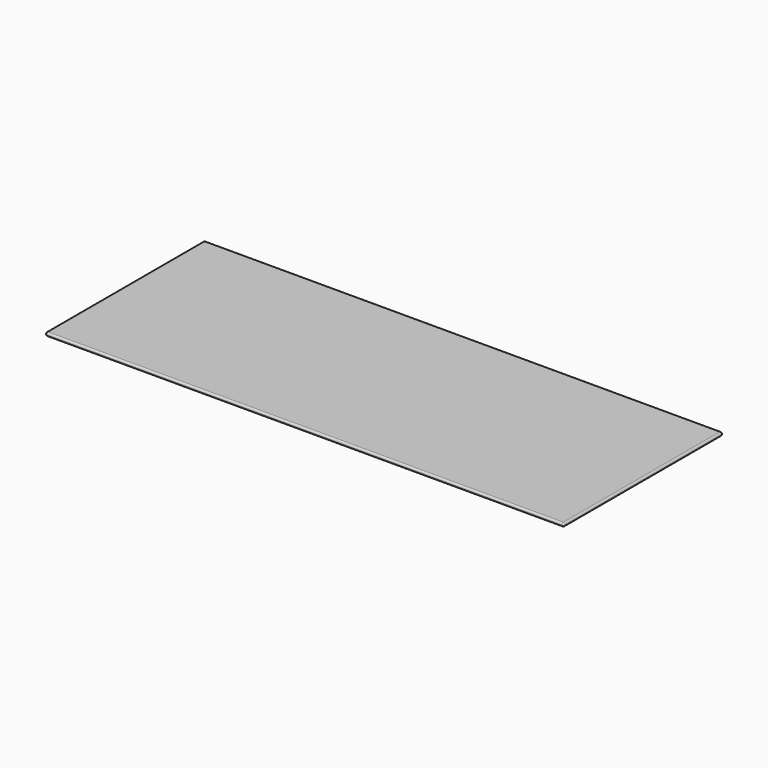
from build123d import *

# Parameters (mm, degrees)
F0_W     = 148.2852
F0_H     = 56.896
F1_DEPTH = 1.016
F2_R     = 0.50799


# Not quite as in the source:
# - a fillet or chamfer is up to 0.001 mm smaller than in the source, because OpenCascade refuses the exact size


with BuildPart() as f1:
    # F0 (on Top) → F1 (new body)
    with BuildSketch(Plane.XY):
        Rectangle(F0_W, F0_H)
    extrude(amount=F1_DEPTH)

    # F2 (radius 0.508 in the source; OpenCascade refuses exactly that, so slightly less here)
    f2_edges = [f1.edges().sort_by_distance(p)[0] for p in [
        (-74.1426, -28.448, 0.508),
        (74.1426, -28.448, 0.508),
        (0, -28.448, 0),
        (0, -28.448, 1.016),
        (-74.1426, 28.448, 0.508),
        (-74.1426, 0, 0),
        (-74.1426, 0, 1.016),
        (74.1426, 28.448, 0.508),
        (0, 28.448, 0),
        (0, 28.448, 1.016),
        (74.1426, 0, 0),
        (74.1426, 0, 1.016),
    ]]
    fillet(f2_edges, radius=F2_R)


solid = f1.part
